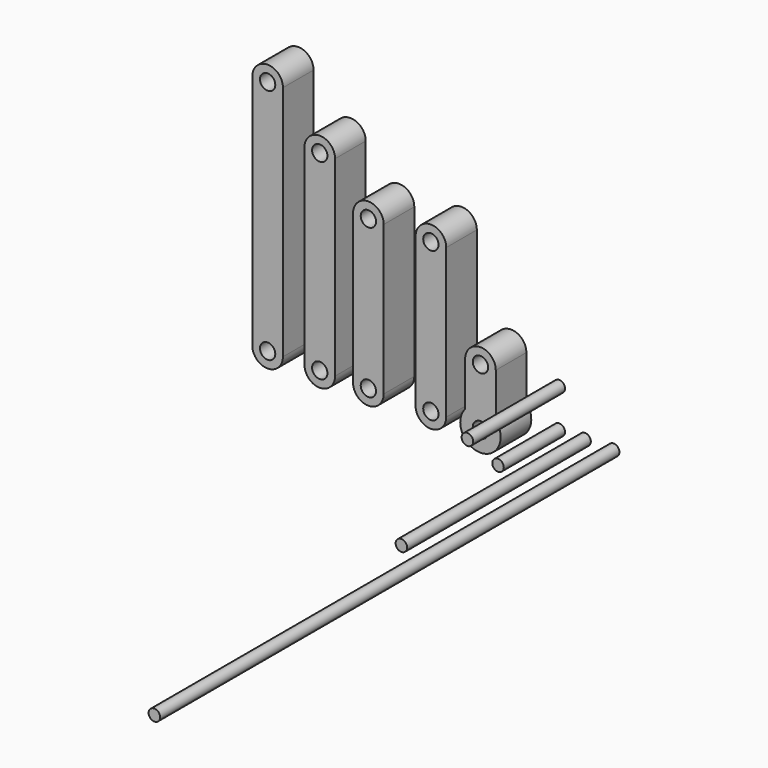
from build123d import *

# Parameters (mm, degrees)
F1_R      = 2
F2_DEPTH  = 10
F3_R      = 2
F4_DEPTH  = 10
F5_R      = 2
F6_DEPTH  = 10
F7_R      = 2
F8_DEPTH  = 10
F9_R      = 2
F10_DEPTH = 10
F11_R     = 1.5
F12_DEPTH = 20
F13_R     = 1.5
F14_DEPTH = 60
F15_DEPTH = 150
F16_R     = 1.5
F17_DEPTH = 30


# Not quite as in the source:
# - a feature names something its author has since deleted; it is built from what else it names


with BuildPart() as f2:
    # F1 (on Front) → F2 (new body)
    with BuildSketch(Plane.XZ):
        with BuildLine():
            Line((-8.5924360901, 3.4478561794), (-8.5924360901, 15))
            ThreePointArc((-8.5924360901, 15), (-12.5924360901, 19), (-16.5924360901, 15))
            Line((-16.5924360901, 15), (-16.5924360901, 3.4478561794))
            ThreePointArc((-16.5924360901, 3.4478561794), (-12.5924360901, -5.2808817667), (-8.5924360901, 3.4478561794))
        make_face()
        with Locations((-12.5924360901, 0)):
            Circle(F1_R, mode=Mode.SUBTRACT)
        with Locations((-12.5924360901, 15)):
            Circle(F1_R, mode=Mode.SUBTRACT)
    extrude(amount=F2_DEPTH)


with BuildPart() as f4:
    # F3 (on Front) → F4 (new body)
    with BuildSketch(Plane.XZ):
        with BuildLine():
            Line((-29.5428169801, 39), (-29.5428169801, 0))
            ThreePointArc((-29.5428169801, 0), (-25.5428169801, -4), (-21.5428169801, 0))
            Line((-21.5428169801, 0), (-21.5428169801, 39))
            ThreePointArc((-21.5428169801, 39), (-25.5428169801, 43), (-29.5428169801, 39))
        make_face()
        with Locations((-25.5428169801, 0)):
            Circle(F3_R, mode=Mode.SUBTRACT)
        with Locations((-25.5428169801, 39)):
            Circle(F3_R, mode=Mode.SUBTRACT)
    extrude(amount=F4_DEPTH)


with BuildPart() as f6:
    # F5 (on Front) → F6 (new body)
    with BuildSketch(Plane.XZ):
        with BuildLine():
            Line((-45.8750046201, 39), (-45.8750046201, 0))
            ThreePointArc((-45.8750046201, 0), (-41.8750046201, -4), (-37.8750046201, 0))
            Line((-37.8750046201, 0), (-37.8750046201, 39))
            ThreePointArc((-37.8750046201, 39), (-41.8750046201, 43), (-45.8750046201, 39))
        make_face()
        with Locations((-41.8750046201, 0)):
            Circle(F5_R, mode=Mode.SUBTRACT)
        with Locations((-41.8750046201, 39)):
            Circle(F5_R, mode=Mode.SUBTRACT)
    extrude(amount=F6_DEPTH)


with BuildPart() as f8:
    # F7 (on Front) → F8 (new body)
    with BuildSketch(Plane.XZ):
        with BuildLine():
            Line((-58.5748284761, 50), (-58.5748284761, 0))
            ThreePointArc((-58.5748284761, 0), (-54.5748284761, -4), (-50.5748284761, 0))
            Line((-50.5748284761, 0), (-50.5748284761, 50))
            ThreePointArc((-50.5748284761, 50), (-54.5748284761, 54), (-58.5748284761, 50))
        make_face()
        with Locations((-54.5748284761, 0)):
            Circle(F7_R, mode=Mode.SUBTRACT)
        with Locations((-54.5748284761, 50)):
            Circle(F7_R, mode=Mode.SUBTRACT)
    extrude(amount=F8_DEPTH)


with BuildPart() as f10:
    # F9 (on Front) → F10 (new body)
    with BuildSketch(Plane.XZ):
        with BuildLine():
            Line((-72.1991949677, 61.9), (-72.1991949677, 0))
            ThreePointArc((-72.1991949677, 0), (-68.1991949677, -4), (-64.1991949677, 0))
            Line((-64.1991949677, 0), (-64.1991949677, 61.9))
            ThreePointArc((-64.1991949677, 61.9), (-68.1991949677, 65.9), (-72.1991949677, 61.9))
        make_face()
        with Locations((-68.1991949677, 0)):
            Circle(F9_R, mode=Mode.SUBTRACT)
        with Locations((-68.1991949677, 61.9)):
            Circle(F9_R, mode=Mode.SUBTRACT)
    extrude(amount=F10_DEPTH)


with BuildPart() as f12:
    # F11 (on Front) → F12 (new body)
    with BuildSketch(Plane.XZ):
        Circle(F11_R)
    extrude(amount=F12_DEPTH)


with BuildPart() as f14:
    # F13 (on Front) → F14 (new body)
    with BuildSketch(Plane.XZ):
        with Locations((6.7503562369, 0)):
            Circle(F13_R)
    extrude(amount=F14_DEPTH)


with BuildPart() as f15:
    # F13 (on Front) → F15 (new body)
    with BuildSketch(Plane.XZ):
        with Locations((14.2067680135, 0)):
            Circle(F13_R)
    extrude(amount=F15_DEPTH)


with BuildPart() as f17:
    # F16 (on Front) → F17 (new body)
    with BuildSketch(Plane.XZ):
        with Locations((0, 10)):
            Circle(F16_R)
    extrude(amount=F17_DEPTH)


solid = Compound([f2.part, f4.part, f6.part, f8.part, f10.part, f12.part, f14.part, f15.part, f17.part])
